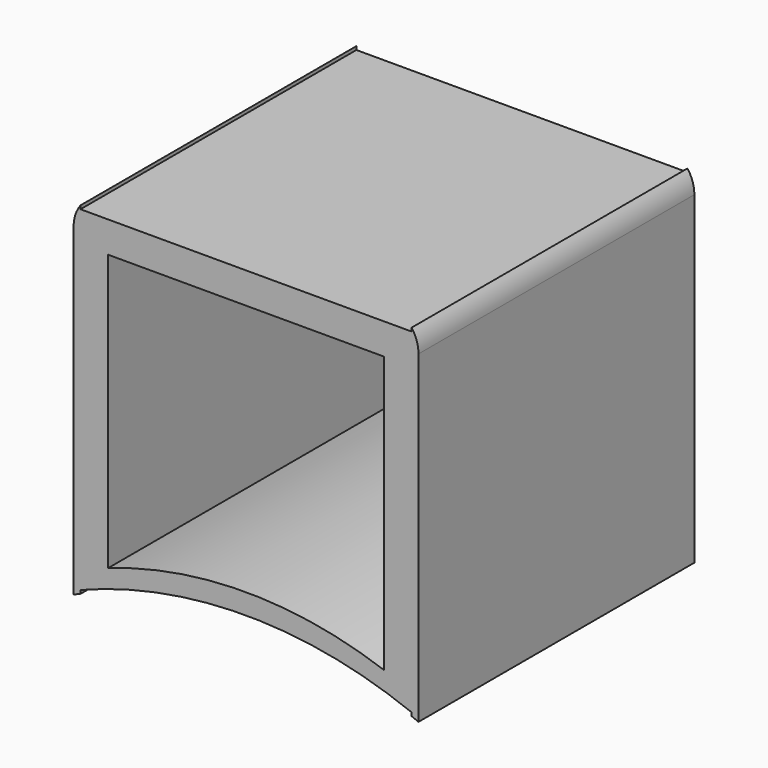
from build123d import *

# Parameters (mm, degrees)
F1_DEPTH    = 50
F2_W        = 48
F2_H        = 0.5
F2_H_2      = 1.5
F3_DEPTH    = 50
F4_T1_DEPTH = 65.1327459504


# Not quite as in the source:
# - a fillet or chamfer that OpenCascade refuses, or shapes differently, is made with other operations: its cross-section is extruded or revolved along the edge and cut away or added


with BuildPart() as f1:
    # F0 (on Front) → F1 (new body)
    with BuildSketch(Plane.XZ):
        with BuildLine():
            Line((25, -25), (25, 25))
            Line((25, 25), (-25, 25))
            Line((-25, 25), (-25, -25))
            ThreePointArc((-25, -25), (0, -20), (25, -25))
        make_face()
        with BuildLine():
            Line((-20, 20), (20, 20))
            Line((20, 20), (20, -20))
            ThreePointArc((20, -20), (0, -16.5685424949), (-20, -20))
            Line((-20, -20), (-20, 20))
        make_face(mode=Mode.SUBTRACT)
    extrude(amount=F1_DEPTH)

    # F2 (on face) → F3 (cut)
    with BuildSketch(Plane.XZ.offset(50)):
        with Locations((0, 24.75)):
            Rectangle(F2_W, F2_H)
        with Locations((0, 25.75)):
            Rectangle(F2_W, F2_H_2)
        with BuildLine():
            Line((-24, -24.0930467578), (-24, -24.5930467578))
            ThreePointArc((-24, -24.5930467578), (0, -20), (24, -24.5930467578))
            Line((24, -24.5930467578), (24, -24.0930467578))
            ThreePointArc((24, -24.0930467578), (0, -19.5376937746), (-24, -24.0930467578))
        make_face()
    extrude(amount=-F3_DEPTH, mode=Mode.SUBTRACT)

    # F4: fillet of radius 5.08 on 2 edges, made by hand

    # F4_s2 → F4_t1 (cut)
    with BuildSketch(Plane.XZ.offset(-7.5663729752)):
        with BuildLine():
            ThreePointArc((25, 21.9734508099), (24.7435256815, 23.567188555), (24, 25))
            Line((24, 25), (25, 25))
            Line((25, 25), (25, 21.9734508099))
        make_face()
        with BuildLine():
            ThreePointArc((-25, 21.9734508099), (-24.7435256815, 23.567188555), (-24, 25))
            Line((-24, 25), (-25, 25))
            Line((-25, 25), (-25, 21.9734508099))
        make_face()
    extrude(amount=F4_T1_DEPTH, mode=Mode.SUBTRACT)


solid = f1.part
